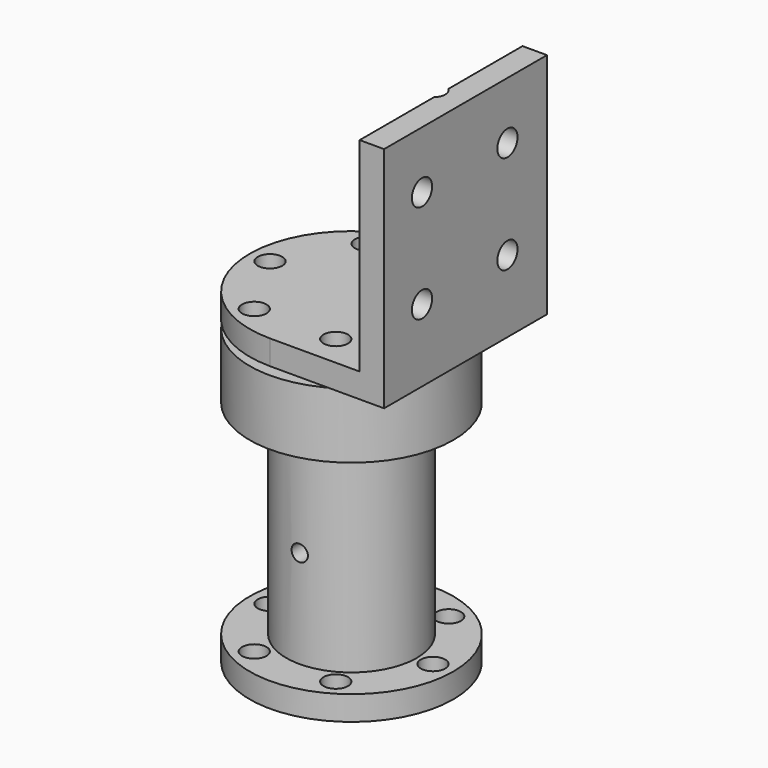
from build123d import *
from build123d import SkipClean  # not in build123d's __all__

# Parameters (mm, degrees)
F0_R      = 12.5
F0_R_2    = 1.5
F1_DEPTH  = 3
F2_R      = 8
F3_DEPTH  = 25
F4_R      = 12.5
F4_R_2    = 8.1
F4_R_3    = 8
F5_DEPTH  = 8
F6_R      = 8.1
F7_DEPTH  = 5
F8_R      = 1
F9_DEPTH  = 40
F10_R     = 3.9
F11_DEPTH = 6
F12_R     = 4.75
F12_R_2   = 3.9
F13_DEPTH = 1.5
F14_R     = 4.75
F14_R_2   = 3.9
F15_DEPTH = 3
F16_DEPTH = 40.001
F18_DEPTH = 25
F19_R     = 1.55
F20_DEPTH = 25


# Not quite as in the source:
# - after a boolean that leaves OpenCascade's solid faulty, fix() repairs it
# - a feature names something its author has since deleted; it is built from what else it names


with BuildPart() as f1:
    # F0 (on Top) → F1 (new body)
    with BuildSketch(Plane.XY):
        Circle(F0_R)
        with Locations((-5, -8.6602540378)):
            Circle(F0_R_2, mode=Mode.SUBTRACT)
        with Locations((5, -8.6602540378)):
            Circle(F0_R_2, mode=Mode.SUBTRACT)
        with Locations((-10, 0)):
            Circle(F0_R_2, mode=Mode.SUBTRACT)
        with Locations((-5, 8.6602540378)):
            Circle(F0_R_2, mode=Mode.SUBTRACT)
        with BuildLine():
            ThreePointArc((2.1, 2.3478713764), (2.8755434269, 1.285982115), (3.15, 0))
            ThreePointArc((3.15, 0), (2.8755434269, -1.285982115), (2.1, -2.3478713764))
            ThreePointArc((2.1, -2.3478713764), (-3.15, 0), (2.1, 2.3478713764))
        make_face(mode=Mode.SUBTRACT)
        with Locations((10, 0)):
            Circle(F0_R_2, mode=Mode.SUBTRACT)
        with Locations((5, 8.6602540378)):
            Circle(F0_R_2, mode=Mode.SUBTRACT)
        with BuildLine():
            ThreePointArc((2.1, -2.3478713764), (2.8755434269, -1.285982115), (3.15, 0))
            ThreePointArc((3.15, 0), (2.8755434269, 1.285982115), (2.1, 2.3478713764))
            Line((2.1, 2.3478713764), (2.1, -2.3478713764))
        make_face()
    extrude(amount=F1_DEPTH)

    # F2 (on face) → F3 (join)
    with BuildSketch(Plane.XY.offset(3)):
        Circle(F2_R)
        with BuildLine():
            Line((2.1, 2.3478713764), (2.1, -2.3478713764))
            ThreePointArc((2.1, -2.3478713764), (-3.15, 0), (2.1, 2.3478713764))
        make_face(mode=Mode.SUBTRACT)
    extrude(amount=F3_DEPTH)

    # F4 (on face) → F5 (join)
    with BuildSketch(Plane.XY.offset(28)):
        Circle(F4_R)
        Circle(F4_R_2, mode=Mode.SUBTRACT)
        Circle(F4_R_2)
        Circle(F4_R_3, mode=Mode.SUBTRACT)
        Circle(F4_R_3)
        with BuildLine():
            ThreePointArc((2.1, -2.3478713764), (-3.15, 0), (2.1, 2.3478713764))
            Line((2.1, 2.3478713764), (2.1, -2.3478713764))
        make_face(mode=Mode.SUBTRACT)
    extrude(amount=F5_DEPTH)

    # F6 (on face) → F7 (cut)
    with BuildSketch(Plane.XY.offset(36)):
        Circle(F6_R)
        with BuildLine():
            ThreePointArc((2.1, -2.3478713764), (-3.15, 0), (2.1, 2.3478713764))
            Line((2.1, 2.3478713764), (2.1, -2.3478713764))
        make_face(mode=Mode.SUBTRACT)
    extrude(amount=-F7_DEPTH, mode=Mode.SUBTRACT)

    # F8 (on Front) → F9 (cut, symmetric)
    with BuildSketch(Plane.XZ):
        with Locations((0, 15)):
            Circle(F8_R)
    extrude(amount=F9_DEPTH, both=True, mode=Mode.SUBTRACT)


with BuildPart() as f11:
    # F10 (on face) → F11 (new body)
    with BuildSketch(Plane.XY.offset(31)):
        Circle(F10_R)
        with BuildLine():
            ThreePointArc((2.1, -2.3478713764), (-3.15, 0), (2.1, 2.3478713764))
            Line((2.1, 2.3478713764), (2.1, -2.3478713764))
        make_face(mode=Mode.SUBTRACT)
        with BuildLine():
            Line((2.1, -2.3478713764), (2.1, 2.3478713764))
            ThreePointArc((2.1, 2.3478713764), (-3.15, 0), (2.1, -2.3478713764))
        make_face()
    extrude(amount=F11_DEPTH)

    # F12 (on face) → F13 (join)
    with BuildSketch(Plane.XY.offset(37)):
        Circle(F12_R)
        Circle(F12_R_2, mode=Mode.SUBTRACT)
        Circle(F12_R_2)
    extrude(amount=-F13_DEPTH)

    # F14 (on face) → F15 (join)
    with BuildSketch(Plane.XY.offset(37)):
        with BuildLine():
            ThreePointArc((0.7329293017, 12.4784940854), (-12.4946223646, 0.3666223758), (0, -12.5))
            ThreePointArc((0, -12.5), (8.8388347648, -8.8388347648), (12.5, 0))
            ThreePointArc((12.5, 0), (9.0942733704, 8.5757910343), (0.7329293017, 12.4784940854))
        make_face()
        Circle(F14_R, mode=Mode.SUBTRACT)
        with BuildLine():
            ThreePointArc((12.5, 0), (8.8388347648, -8.8388347648), (0, -12.5))
            Line((0, -12.5), (14, -12.5))
            Line((14, -12.5), (14, 12.4784940854))
            Line((14, 12.4784940854), (0.7329293017, 12.4784940854))
            ThreePointArc((0.7329293017, 12.4784940854), (9.0942733704, 8.5757910343), (12.5, 0))
        make_face()
        Circle(F14_R)
        Circle(F14_R_2, mode=Mode.SUBTRACT)
        Circle(F14_R_2)
    extrude(amount=F15_DEPTH)

    # F0 (on Top) → F16 (cut, through all)
    with BuildSketch(Plane.XY):
        with Locations((-5, 8.6602540378)):
            Circle(F0_R_2)
        with Locations((5, 8.6602540378)):
            Circle(F0_R_2)
        with Locations((10, 0)):
            Circle(F0_R_2)
        with Locations((5, -8.6602540378)):
            Circle(F0_R_2)
        with Locations((-5, -8.6602540378)):
            Circle(F0_R_2)
        with Locations((-10, 0)):
            Circle(F0_R_2)
    extrude(amount=F16_DEPTH, mode=Mode.SUBTRACT)

    # F17 (on face) → F18 (join)
    with BuildSketch(Plane.XY.offset(40)):
        with BuildLine():
            Line((11, -12.5), (14, -12.5))
            Line((14, -12.5), (14, 12.4784940854))
            Line((14, 12.4784940854), (11, 12.4784940854))
            Line((11, 12.4784940854), (11, 1.1180339887))
            ThreePointArc((11, 1.1180339887), (11.3693063938, 0.6123724357), (11.5, 0))
            ThreePointArc((11.5, 0), (11.3693063938, -0.6123724357), (11, -1.1180339887))
            Line((11, -1.1180339887), (11, -12.5))
        make_face()
    with SkipClean():  # cleaning this boolean's faces spoils the solid; the shape is the same uncleaned
        extrude(amount=F18_DEPTH)

    # F19 (on face) → F20 (cut)
    with BuildSketch(Plane(origin=(11, 0, 0), x_dir=(0, -1, 0), z_dir=(-1, 0, 0))):
        with Locations((-6.413962692, 45.8764471114)):
            Circle(F19_R)
        with Locations((-6.413962692, 57.9764471114)):
            Circle(F19_R)
        with Locations((6.686037308, 45.8764471114)):
            Circle(F19_R)
        with Locations((6.686037308, 57.9764471114)):
            Circle(F19_R)
    extrude(amount=-F20_DEPTH, mode=Mode.SUBTRACT)

    add(f11.part.fix(), mode=Mode.REPLACE)


solid = Compound([f1.part, f11.part])
